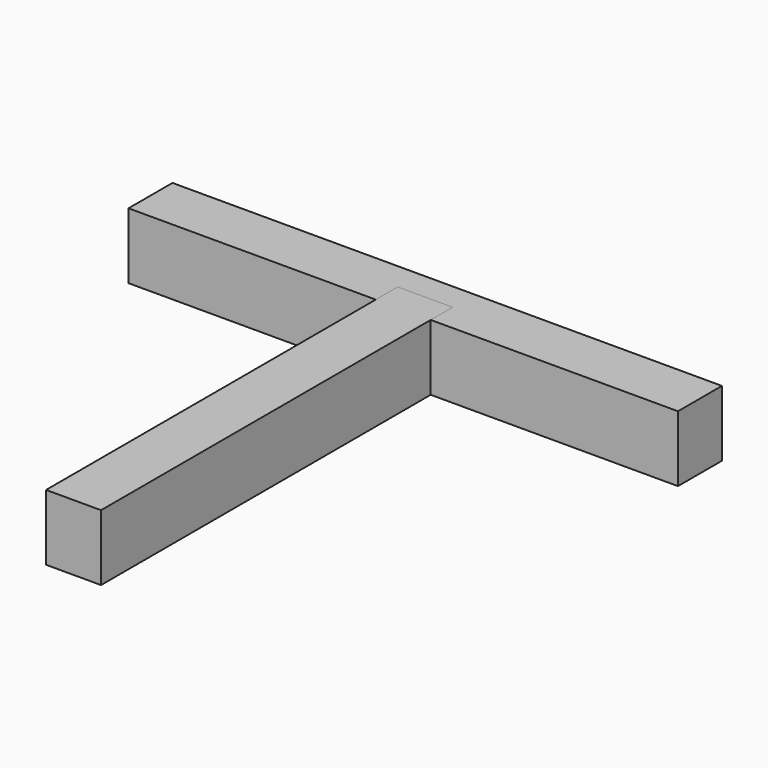
from build123d import *

# Parameters (mm, degrees)
F0_W     = 2540
F0_H     = 254
F1_DEPTH = 304.8
F2_W     = 254
F2_H     = 127
F3_DEPTH = 152.4
F4_W     = 254
F4_H     = 2032
F5_DEPTH = 304.8
F6_W     = 254
F6_H     = 152.4
F7_DEPTH = 127


with BuildPart() as f1:
    # F0 (on Top) → F1 (new body)
    with BuildSketch(Plane.XY):
        with Locations((0, 127)):
            Rectangle(F0_W, F0_H)
    extrude(amount=F1_DEPTH)

    # F2 (on face) → F3 (cut)
    with BuildSketch(Plane.XY.offset(304.8)):
        with Locations((0, 63.5)):
            Rectangle(F2_W, F2_H)
    extrude(amount=-F3_DEPTH, mode=Mode.SUBTRACT)


with BuildPart() as f5:
    # F4 (on Top) → F5 (new body)
    with BuildSketch(Plane.XY):
        with Locations((0, -889)):
            Rectangle(F4_W, F4_H)
    extrude(amount=F5_DEPTH)

    # F6 (on face) → F7 (cut)
    with BuildSketch(Plane(origin=(0, 127, 0), x_dir=(-1, 0, 0), z_dir=(0, 1, 0))):
        with Locations((0, 76.2)):
            Rectangle(F6_W, F6_H)
    extrude(amount=-F7_DEPTH, mode=Mode.SUBTRACT)


solid = Compound([f1.part, f5.part])
